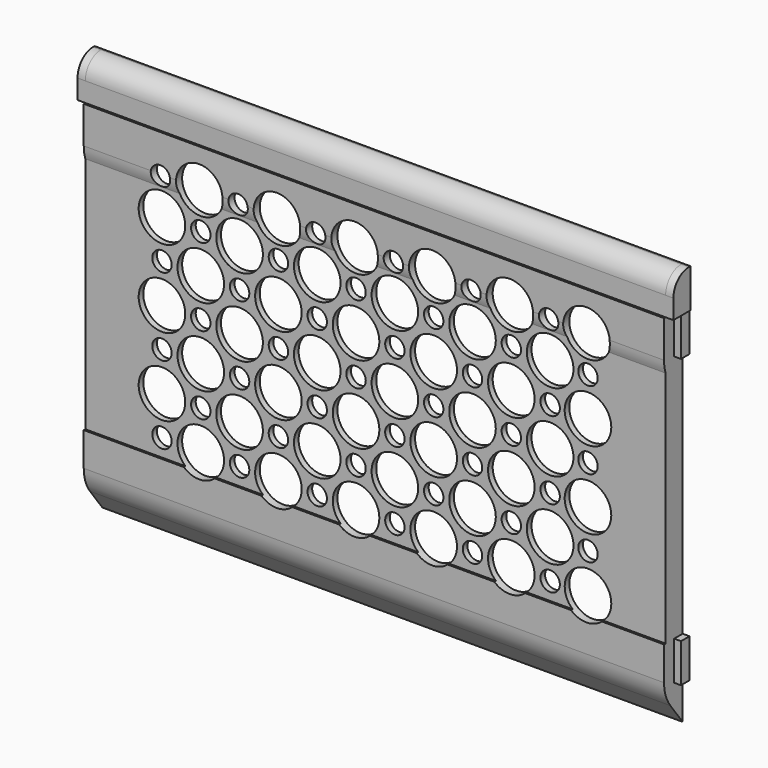
from build123d import *

# Parameters (mm, degrees)
F1_DEPTH    = 149.5
F2_W        = 2.75
F2_H        = 10
F3_DEPTH    = 1.75
F4_W        = 2.75
F4_H        = 10
F5_DEPTH    = 1.75
F6_R        = 5
F7_T1_DEPTH = 161.7791616627
F7_T3_DEPTH = 166.1666666667
F8_W        = 129.5
F8_H        = 79
F9_DEPTH    = 25
F11_DEPTH   = 129.5
F13_D       = 12
F13_DEPTH   = 12
F13_TIP     = 3.6051637142
F14_D       = 5
F14_DEPTH   = 12
F14_TIP     = 1.5021515476
F16_DEPTH   = 2
F18_DEPTH   = 2


# Not quite as in the source:
# - a fillet or chamfer that OpenCascade refuses, or shapes differently, is made with other operations: its cross-section is extruded or revolved along the edge and cut away or added


with BuildPart() as f1:
    # F0 (on Right) → F1 (new body)
    with BuildSketch(Plane.YZ):
        Polygon((5.5, 38.1918546259), (5.5, 58.1918546259), (0, 58.1918546259), (0, 48.1918546259), (2.5, 48.1918546259), (2.5, 38.1918546259), align=None)
        Polygon((5.5, 28.1918546259), (5.5, 38.1918546259), (2.5, 38.1918546259), (2.5, 48.1918546259), (0, 48.1918546259), (0, 35.5251879593), align=None)
        Polygon((5.5, -35.8081453741), (5.5, 28.1918546259), (0, 35.5251879593), (0, -25.8081453741), (2.5, -25.8081453741), (2.5, -35.8081453741), align=None)
        Polygon((5.5, -45.8081453741), (5.5, -35.8081453741), (2.5, -35.8081453741), (2.5, -25.8081453741), (0, -25.8081453741), (0, -38.4748120407), align=None)
        Polygon((0, 35.5251879593), (0, 48.1918546259), (-0.5, 48.1918546259), (-0.5, 36.1918546259), align=None)
        Polygon((0, -38.4748120407), (0, -25.8081453741), (-0.5, -25.8081453741), (-0.5, -37.8081453741), align=None)
    extrude(amount=-F1_DEPTH)

    # F2 (on face) → F3 (join)
    with BuildSketch(Plane(origin=(-149.5, 0, 0), x_dir=(0, -1, 0), z_dir=(-1, 0, 0))):
        with Locations((-4.125, 43.1918546259)):
            Rectangle(F2_W, F2_H)
        with Locations((-4.125, -30.8081453741)):
            Rectangle(F2_W, F2_H)
    extrude(amount=F3_DEPTH)

    # F4 (on face) → F5 (join)
    with BuildSketch(Plane.YZ):
        with Locations((4.125, -30.8081453741)):
            Rectangle(F4_W, F4_H)
        with Locations((4.125, 43.1918546259)):
            Rectangle(F4_W, F4_H)
    extrude(amount=F5_DEPTH)

    # F6
    f6_edges = [f1.edges().sort_by_distance(p)[0] for p in [
        (-74.75, 0, 58.191855),
    ]]
    fillet(f6_edges, radius=F6_R)

    # F7: fillet of radius 10 on 2 edges, made by hand

    # F7_s2 → F7_t1 (cut)
    with BuildSketch(Plane.YZ.offset(-155.6395808313)):
        with BuildLine():
            ThreePointArc((-0.5, 38.6476869585), (-0.3742088291, 37.0665481284), (0, 35.5251879593))
            Line((0, 35.5251879593), (-0.5, 36.1918546259))
            Line((-0.5, 36.1918546259), (-0.5, 38.6476869585))
        make_face()
    extrude(amount=F7_T1_DEPTH, mode=Mode.SUBTRACT)

    # F7_s4 → F7_t3 (cut)
    with BuildSketch(Plane.YZ.offset(-157.8333333333)):
        with BuildLine():
            ThreePointArc((-0.5, -34.4748120407), (0.0131670195, -37.6370897009), (1.5, -40.4748120407))
            Line((1.5, -40.4748120407), (-0.5, -37.8081453741))
            Line((-0.5, -37.8081453741), (-0.5, -34.4748120407))
        make_face()
    extrude(amount=F7_T3_DEPTH, mode=Mode.SUBTRACT)

    # F8 (on face) → F9 (cut)
    with BuildSketch(Plane(origin=(0, 5.5, 0), x_dir=(-1, 0, 0), z_dir=(0, 1, 0))):
        with Locations((74.75, 8.6918546259)):
            Rectangle(F8_W, F8_H)
    extrude(amount=-F9_DEPTH, mode=Mode.SUBTRACT)

    # F10 (on face) → F11 (join)
    with BuildSketch(Plane.YZ.offset(-139.5)):
        with BuildLine():
            Line((1.5, -30.8081453741), (1.5, 48.1918546259))
            Line((1.5, 48.1918546259), (0, 48.1918546259))
            Line((0, 48.1918546259), (-0.5, 48.1918546259))
            Line((-0.5, 48.1918546259), (-0.5, 38.6476869585))
            ThreePointArc((-0.5, 38.6476869585), (-0.3742088291, 37.0665481284), (0, 35.5251879593))
            Line((0, 35.5251879593), (0, -25.8081453741))
            Line((0, -25.8081453741), (-0.5, -25.8081453741))
            Line((-0.5, -25.8081453741), (-0.5, -30.8081453741))
            Line((-0.5, -30.8081453741), (1.5, -30.8081453741))
        make_face()
    extrude(amount=F11_DEPTH)

    # F13
    with Locations(Plane(origin=(0, 1.5, 0), x_dir=(-1, 0, 0), z_dir=(0, 1, 0))):
        with Locations((20, -21.3081453741), (39.75, -21.3081453741), (59.75, -21.3081453741), (79.75, -21.3081453741), (99.75, -21.3081453741), (119.75, -21.3081453741), (129.75, -11.3081453741), (109.75, -11.3081453741), (89.75, -11.3081453741), (69.75, -11.3081453741), (49.75, -11.3081453741), (29.75, -11.3081453741), (20, -1.3081453741), (39.75, -1.3081453741), (59.75, -1.3081453741), (79.75, -1.3081453741), (99.75, -1.3081453741), (119.75, -1.3081453741), (129.75, 8.6918546259), (109.75, 8.6918546259), (89.75, 8.6918546259), (69.75, 8.6918546259), (49.75, 8.6918546259), (29.75, 8.6918546259), (20, 18.6918546259), (39.75, 18.6918546259), (59.75, 18.6918546259), (79.75, 18.6918546259), (99.75, 18.6918546259), (119.75, 18.6918546259), (129.75, 28.6918546259), (109.75, 28.6918546259), (89.75, 28.6918546259), (69.75, 28.6918546259), (49.75, 28.6918546259), (29.75, 28.6918546259), (20, 38.1918546259), (39.75, 38.1918546259), (59.75, 38.1918546259), (79.75, 38.1918546259), (99.75, 38.1918546259), (119.75, 38.1918546259)):
            Hole(F13_D / 2, depth=F13_DEPTH)
            with Locations((0, 0, -(F13_DEPTH + F13_TIP / 2))):  # 118° drill point
                Cone(0, F13_D / 2, F13_TIP, mode=Mode.SUBTRACT)

    # F14
    with Locations(Plane(origin=(0, 1.5, 0), x_dir=(-1, 0, 0), z_dir=(0, 1, 0))):
        with Locations((29.75, 38.1918546259), (49.75, 38.1918546259), (69.75, 38.1918546259), (89.75, 38.1918546259), (109.75, 38.1918546259), (129.75, 38.1918546259), (119.75, 28.6918546259), (99.75, 28.6918546259), (79.75, 28.6918546259), (59.75, 28.6918546259), (39.75, 28.6918546259), (20, 28.6918546259), (29.75, 18.6918546259), (49.75, 18.6918546259), (69.75, 18.6918546259), (89.75, 18.6918546259), (109.75, 18.6918546259), (129.75, 18.6918546259), (119.75, 8.6918546259), (99.75, 8.6918546259), (79.75, 8.6918546259), (59.75, 8.6918546259), (39.75, 8.6918546259), (20, 8.6918546259), (29.75, -1.3081453741), (49.75, -1.3081453741), (69.75, -1.3081453741), (89.75, -1.3081453741), (109.75, -1.3081453741), (129.75, -1.3081453741), (119.75, -11.3081453741), (99.75, -11.3081453741), (79.75, -11.3081453741), (59.75, -11.3081453741), (39.75, -11.3081453741), (20, -11.3081453741), (29.75, -21.3081453741), (49.75, -21.3081453741), (69.75, -21.3081453741), (89.75, -21.3081453741), (109.75, -21.3081453741), (129.75, -21.3081453741)):
            Hole(F14_D / 2, depth=F14_DEPTH)
            with Locations((0, 0, -(F14_DEPTH + F14_TIP / 2))):  # 118° drill point
                Cone(0, F14_D / 2, F14_TIP, mode=Mode.SUBTRACT)

    # F15 (on face) → F16 (join)
    with BuildSketch(Plane(origin=(-149.5, 0, 0), x_dir=(0, -1, 0), z_dir=(-1, 0, 0))):
        with BuildLine():
            Line((-5.5, 48.1918546259), (-2.75, 48.1918546259))
            Line((-2.75, 48.1918546259), (0, 48.1918546259))
            Line((0, 48.1918546259), (0, 53.1918546259))
            ThreePointArc((0, 53.1918546259), (-1.4644660941, 56.7273885319), (-5, 58.1918546259))
            Line((-5, 58.1918546259), (-5.5, 58.1918546259))
            Line((-5.5, 58.1918546259), (-5.5, 48.1918546259))
        make_face()
    extrude(amount=F16_DEPTH)

    # F17 (on face) → F18 (join)
    with BuildSketch(Plane.YZ):
        with BuildLine():
            Line((0, 48.1918546259), (2.75, 48.1918546259))
            Line((2.75, 48.1918546259), (5.5, 48.1918546259))
            Line((5.5, 48.1918546259), (5.5, 58.1918546259))
            Line((5.5, 58.1918546259), (5, 58.1918546259))
            ThreePointArc((5, 58.1918546259), (1.4644660941, 56.7273885319), (0, 53.1918546259))
            Line((0, 53.1918546259), (0, 48.1918546259))
        make_face()
    extrude(amount=F18_DEPTH)


solid = f1.part
